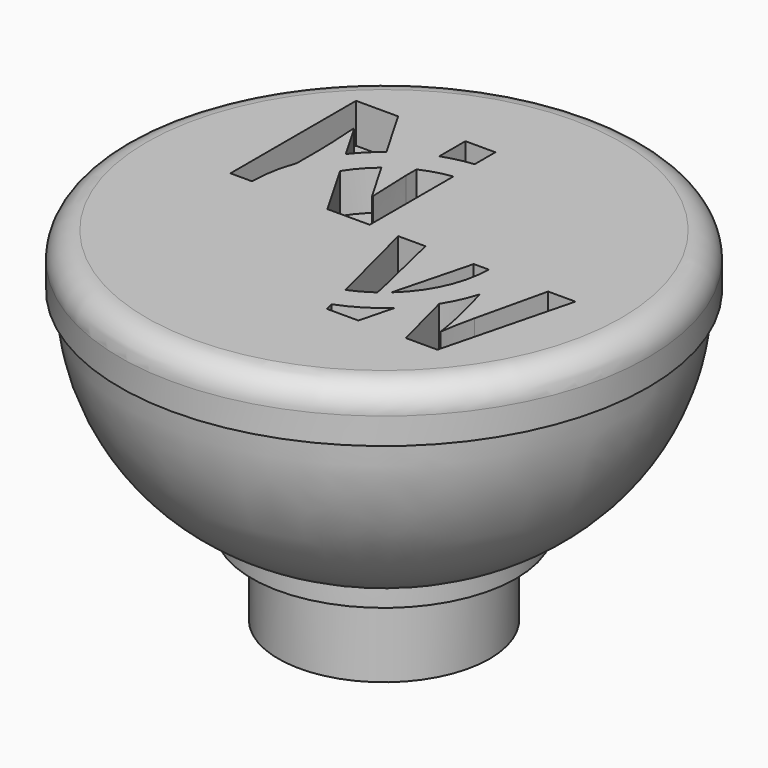
from build123d import *

# Parameters (mm, degrees)
F0_R           = 4
F1_DEPTH       = 13
F0_R_2         = 10
F0_R_3         = 5
F2_DEPTH       = 2
F3_R           = 1
F4_TEXT_SIZE   = 8.3333333333
F4_TEXT_SIZE_2 = 6.9444444444
F5_DEPTH       = 1.5
F7_DEPTH       = 10


# Not quite as in the source:
# - Text() gives the source's letters only with a copy of the font that has no kerning and outlines rounded to 1/6400 em; it was checked with that copy


with BuildPart() as f1:
    # F0 (on Top) → F1 (new body)
    with BuildSketch(Plane.XY):
        Circle(F0_R)
    extrude(amount=-F1_DEPTH)

    # F0 (on Top) → F2 (join)
    with BuildSketch(Plane.XY):
        Circle(F0_R_2)
        Circle(F0_R_3, mode=Mode.SUBTRACT)
        Circle(F0_R_3)
        Circle(F0_R, mode=Mode.SUBTRACT)
    extrude(amount=-F2_DEPTH)

    # F3
    f3_edges = [f1.edges().sort_by_distance(p)[0] for p in [
        (-10, 0, 0),
    ]]
    fillet(f3_edges, radius=F3_R)

    # F4 (on Top) + F0 (on Top) → F5 (cut)
    with BuildSketch(Plane.XY):
        with Locations((-6.56640625, 0)):
            Text('N', F4_TEXT_SIZE, font='Open Sans', font_style=FontStyle.BOLD, text_align=(TextAlign.LEFT, TextAlign.BOTTOM))
        with Locations((0.5710121205, -5)):
            Text('W', F4_TEXT_SIZE_2, font='Open Sans', font_style=FontStyle.BOLD, text_align=(TextAlign.LEFT, TextAlign.BOTTOM))
    with BuildSketch(Plane.XY):
        Circle(F0_R_3)
        Circle(F0_R, mode=Mode.SUBTRACT)
    extrude(amount=-F5_DEPTH, mode=Mode.SUBTRACT)

    # F0 (on Top) → F7 (join)
    with BuildSketch(Plane.XY):
        Circle(F0_R_3)
        Circle(F0_R, mode=Mode.SUBTRACT)
    extrude(amount=-F7_DEPTH)

    # F6 (on Front) → F8 (revolve)
    with BuildSketch(Plane.XZ):
        with BuildLine():
            Line((9.7065037116, -1.5558530577), (0, -1.5558530577))
            Line((0, -1.5558530577), (0, -9.9336309358))
            ThreePointArc((0, -9.9336309358), (6.8969412096, -8.1125629854), (9.7065037116, -1.5558530577))
        make_face()
    revolve(axis=Axis((0, 0, -4.9668154679), (0, 0, -1)))


solid = f1.part
